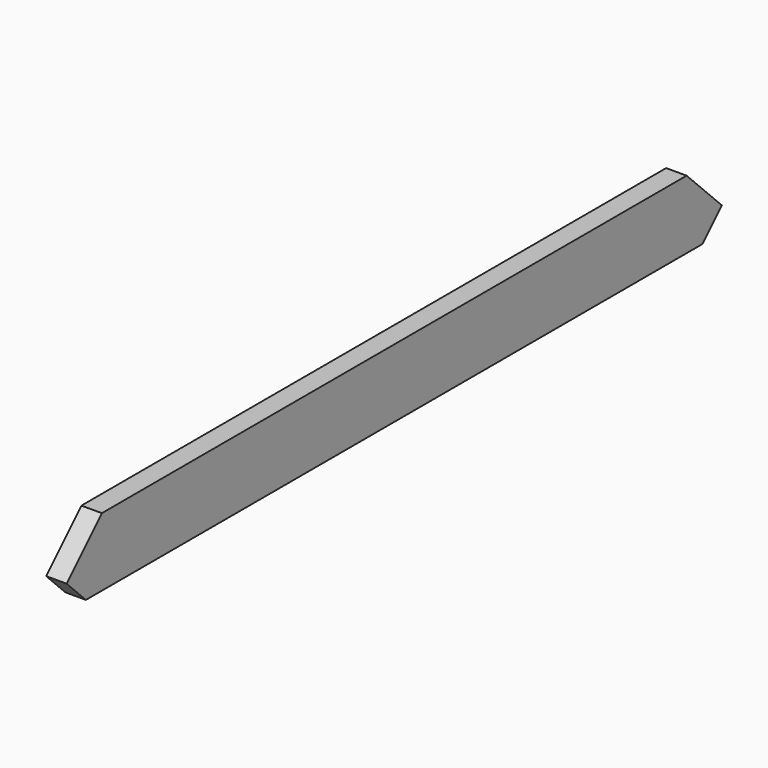
from build123d import *

# Parameters (mm, degrees)
F0_W     = 19.05
F0_H     = 63.5
F1_DEPTH = 762
F2_SIZE  = 41.0464
F7_DEPTH = 19.051
F8_SIZE  = 22.45359


# Not quite as in the source:
# - a fillet or chamfer is up to 0.001 mm smaller than in the source, because OpenCascade refuses the exact size


with BuildPart() as f1:
    # F0 (on Front) → F1 (new body)
    with BuildSketch(Plane.XZ):
        with Locations((9.525, -31.75)):
            Rectangle(F0_W, F0_H)
    extrude(amount=F1_DEPTH)

    # F2
    f2_edges = [f1.edges().sort_by_distance(p)[0] for p in [
        (9.525, 0, 0),
        (9.525, -762, 0),
    ]]
    chamfer(f2_edges, length=F2_SIZE)

    # F6 (on face) → F7 (cut, through all)
    with BuildSketch(Plane(origin=(0, 0, 0), x_dir=(0, -1, 0), z_dir=(-1, 0, 0))):
        Polygon((0, -41.0493596973), (0, -63.5), (22.4506403027, -63.5), align=None)
    extrude(amount=-F7_DEPTH, mode=Mode.SUBTRACT)

    # F8 (size 22.4536 in the source; OpenCascade refuses exactly that, so slightly less here)
    f8_edges = [f1.edges().sort_by_distance(p)[0] for p in [
        (9.525, -762, -63.5),
    ]]
    chamfer(f8_edges, length=F8_SIZE)


solid = f1.part
